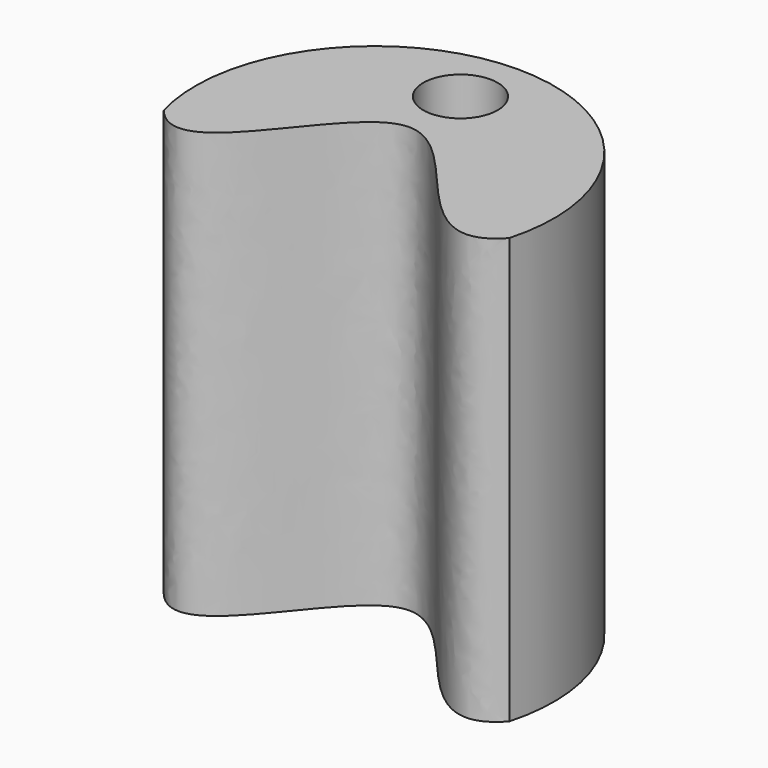
from build123d import *

# Parameters (mm, degrees)
F1_DEPTH = 25.4
F2_R     = 2.2195966307
F3_DEPTH = 22.225
F4_T     = 2.54


# Not quite as in the source:
# - a shell that OpenCascade refuses in one call is made with other operations: the cavity is built on its own and cut out


with BuildPart() as f1:
    # F0 (on Top) → F1 (new body)
    with BuildSketch(Plane.XY):
        with BuildLine():
            add(Edge.make_bspline(
                [(-9.9282488227, 0), (-6.6706539696, -3.9497121754), (-0.009677335, 15.6506770315), (7.0833598277, -4.0324827548), (10.7069341466, 0)],
                knots=[0, 0, 0, 0, 0.4928486408, 1, 1, 1, 1], degree=3))
            ThreePointArc((10.7069341466, 0), (0.3893426619, 13.5539694573), (-9.9282488227, 0))
        make_face()
    extrude(amount=F1_DEPTH)

    # F2 (on face) → F3 (cut)
    with BuildSketch(Plane.XY.offset(25.4)):
        with Locations((0, 9.7335772589)):
            Circle(F2_R)
    extrude(amount=-F3_DEPTH, mode=Mode.SUBTRACT)

    # F4: shell of thickness 2.54, made by hand


with BuildPart() as f4_core1:
    # F4_t2: copy of F1
    add(f1.part)

    # the walls: a layer under each face that stays
    f4_faces = [f4_core1.faces().sort_by_distance(p)[0] for p in [
        (0.1475396024, 5.8275524101, 12.7),
        (0.3893426619, 13.5539694573, 12.7),
        (0.3893426619, 5.8090971383, 0),
        (0.3893426619, 5.8090971383, 25.4),
        (-2.2195966307, 9.7335772589, 14.2875),
        (0, 9.7335772589, 3.175),
    ]]
    thicken(f4_faces, amount=-F4_T, mode=Mode.SUBTRACT)

    # F4_s3 → F4_t4 (revolve, cut)
    with BuildSketch(Plane.XZ.offset(-9.7335772589)):
        Polygon((2.1941966307, 3.2004), (4.7595966307, 3.175), (4.7595966307, 0.635), (2.2195966307, 0.635), align=None)
    revolve(axis=Axis((0, 9.7335772589, 3.175), (0, 0, 1)), mode=Mode.SUBTRACT)


with BuildPart() as f1_1:
    add(f1.part)

    # what is left inside the walls is the cavity
    f4_cavity = [f4_core1.part.solids().sort_by_distance(p)[0] for p in [
        (-7.093674, 6.050134, 16.086667),
        (7.742605, 6.337968, 16.086667),
    ]]
    add(f4_cavity, mode=Mode.SUBTRACT)


solid = f1_1.part
